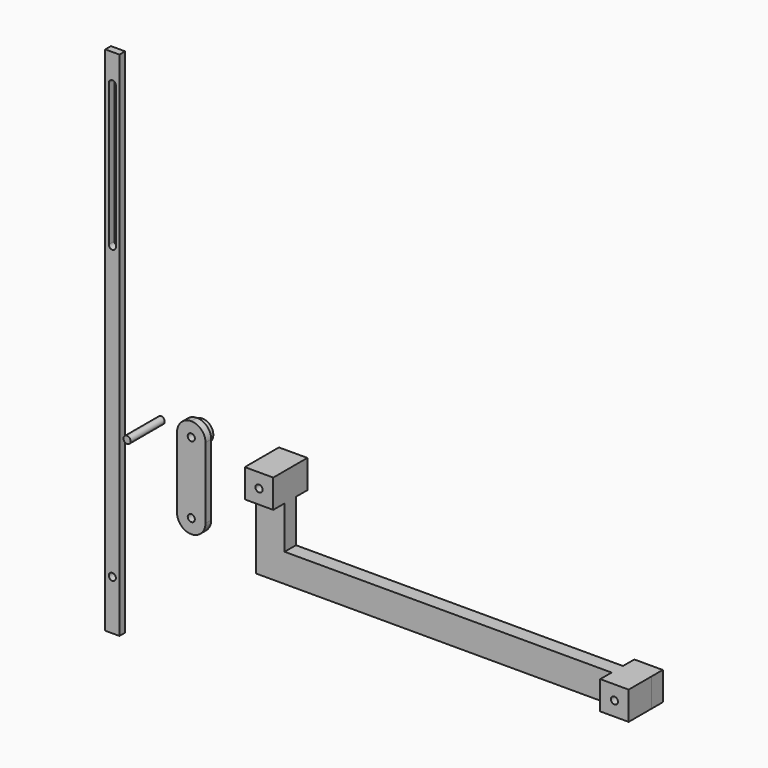
from build123d import *

# Parameters (mm, degrees)
F0_R          = 0.5
F1_DEPTH      = 2
F2_DEPTH      = 2
F3_DEPTH      = 2
F4_DEPTH      = 4
F4_DEPTH_BACK = 2
F5_R          = 1.5
F5_R_2        = 0.5
F6_DEPTH      = 1
F7_DEPTH      = 1
F8_R          = 0.5
F9_DEPTH      = 6
F10_W         = 2
F10_H         = 72
F10_R         = 0.5
F11_DEPTH     = 1


with BuildPart() as f1:
    # F0 (on Front) → F1 (new body)
    with BuildSketch(Plane.XZ):
        Polygon((-2, 0), (0, 0), (2, 0), (48, 0), (48, 4), (2, 4), (2, 10), (-2, 10), align=None)
        Polygon((48, 4), (48, 0), (50, 0), (52, 0), (52, 4), (50, 4), align=None)
        with Locations((50, 2)):
            Circle(F0_R, mode=Mode.SUBTRACT)
        Polygon((-2, 12), (-2, 10), (2, 10), (2, 12), (2, 14), (-2, 14), align=None)
        with Locations((0, 12)):
            Circle(F0_R, mode=Mode.SUBTRACT)
    extrude(amount=F1_DEPTH)

    # F0 (on Front) → F2 (join)
    with BuildSketch(Plane.XZ):
        Polygon((-2, 12), (-2, 10), (2, 10), (2, 12), (2, 14), (-2, 14), align=None)
        with Locations((0, 12)):
            Circle(F0_R, mode=Mode.SUBTRACT)
        Polygon((48, 4), (48, 0), (50, 0), (52, 0), (52, 4), (50, 4), align=None)
        with Locations((50, 2)):
            Circle(F0_R, mode=Mode.SUBTRACT)
    extrude(amount=-F2_DEPTH)


with BuildPart() as f3:
    # F0 (on Front) → F3 (new body)
    with BuildSketch(Plane.XZ):
        Polygon((-2, 0), (0, 0), (2, 0), (48, 0), (48, 4), (2, 4), (2, 10), (-2, 10), align=None)
        Polygon((48, 4), (48, 0), (50, 0), (52, 0), (52, 4), (50, 4), align=None)
        with Locations((50, 2)):
            Circle(F0_R, mode=Mode.SUBTRACT)
        Polygon((-2, 12), (-2, 10), (2, 10), (2, 12), (2, 14), (-2, 14), align=None)
        with Locations((0, 12)):
            Circle(F0_R, mode=Mode.SUBTRACT)
    extrude(amount=F3_DEPTH)

    # F0 (on Front) → F4 (join, two sides)
    with BuildSketch(Plane.XZ) as f4_sk:
        Polygon((-2, 12), (-2, 10), (2, 10), (2, 12), (2, 14), (-2, 14), align=None)
        with Locations((0, 12)):
            Circle(F0_R, mode=Mode.SUBTRACT)
        Polygon((48, 4), (48, 0), (50, 0), (52, 0), (52, 4), (50, 4), align=None)
        with Locations((50, 2)):
            Circle(F0_R, mode=Mode.SUBTRACT)
    extrude(amount=F4_DEPTH)
    extrude(f4_sk.sketch, amount=-F4_DEPTH_BACK)


with BuildPart() as f6:
    # F5 (on Front) → F6 (new body)
    with BuildSketch(Plane.XZ):
        with BuildLine():
            ThreePointArc((-11.9296857071, 15.2392054426), (-13.3438992695, 14.653419005), (-13.9296857071, 13.2392054426))
            Line((-13.9296857071, 13.2392054426), (-13.9296857071, 8.2392054426))
            Line((-13.9296857071, 8.2392054426), (-9.9296857071, 8.2392054426))
            Line((-9.9296857071, 8.2392054426), (-9.9296857071, 13.2392054426))
            ThreePointArc((-9.9296857071, 13.2392054426), (-10.5154721447, 14.653419005), (-11.9296857071, 15.2392054426))
        make_face()
        with Locations((-11.9296857071, 13.2392054426)):
            Circle(F5_R, mode=Mode.SUBTRACT)
        with BuildLine():
            Line((-9.9296857071, 8.2392054426), (-13.9296857071, 8.2392054426))
            Line((-13.9296857071, 8.2392054426), (-13.9296857071, 3.2392054426))
            ThreePointArc((-13.9296857071, 3.2392054426), (-13.3438992695, 1.8249918802), (-11.9296857071, 1.2392054426))
            ThreePointArc((-11.9296857071, 1.2392054426), (-10.5154721447, 1.8249918802), (-9.9296857071, 3.2392054426))
            Line((-9.9296857071, 3.2392054426), (-9.9296857071, 8.2392054426))
        make_face()
        with Locations((-11.9296857071, 3.2392054426)):
            Circle(F5_R, mode=Mode.SUBTRACT)
        with Locations((-11.9296857071, 3.2392054426)):
            Circle(F5_R)
        with Locations((-11.9296857071, 3.2392054426)):
            Circle(F5_R_2, mode=Mode.SUBTRACT)
        with Locations((-11.9296857071, 13.2392054426)):
            Circle(F5_R)
        with Locations((-11.9296857071, 13.2392054426)):
            Circle(F5_R_2, mode=Mode.SUBTRACT)
    extrude(amount=F6_DEPTH)

    # F5 (on Front) → F7 (join)
    with BuildSketch(Plane.XZ):
        with Locations((-11.9296857071, 13.2392054426)):
            Circle(F5_R)
        with Locations((-11.9296857071, 13.2392054426)):
            Circle(F5_R_2, mode=Mode.SUBTRACT)
    extrude(amount=-F7_DEPTH)


with BuildPart() as f9:
    # F8 (on Front) → F9 (new body)
    with BuildSketch(Plane.XZ):
        with Locations((-16.9640984386, 13.3190788329)):
            Circle(F8_R)
    extrude(amount=F9_DEPTH)


with BuildPart() as f11:
    # F10 (on Front) → F11 (new body)
    with BuildSketch(Plane.XZ):
        with Locations((-23.035446647, 21.3490054011)):
            Rectangle(F10_W, F10_H)
        with Locations((-23.035446647, -7.6509945989)):
            Circle(F10_R, mode=Mode.SUBTRACT)
        with BuildLine():
            ThreePointArc((-22.535446647, 33.3490054011), (-23.035446647, 32.8490054011), (-23.535446647, 33.3490054011))
            Line((-23.535446647, 33.3490054011), (-23.535446647, 53.3490054011))
            ThreePointArc((-23.535446647, 53.3490054011), (-23.035446647, 53.8490054011), (-22.535446647, 53.3490054011))
            Line((-22.535446647, 53.3490054011), (-22.535446647, 33.3490054011))
        make_face(mode=Mode.SUBTRACT)
    extrude(amount=F11_DEPTH)


solid = Compound([f1.part, f3.part, f6.part, f9.part, f11.part])
